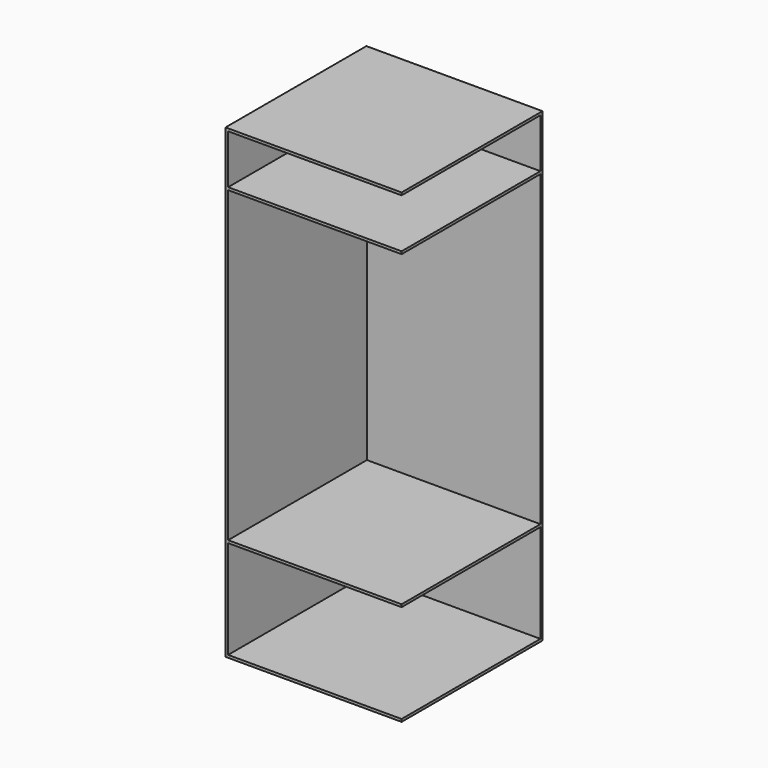
from build123d import *

# Parameters (mm, degrees)
F0_W        = 167.5
F0_H        = 85
F0_W_2      = 2.5
F0_H_2      = 2.5
F0_H_3      = 82.5
F1_DEPTH    = 100
F2_T        = -2.5
F3_W        = 2.5
F3_H        = 167.5
F3_W_2      = 167.5
F3_H_2      = 2.5
F4_DEPTH    = 300
F5_T        = 2.5
F5_T3_DEPTH = 172.5
F5_T5_DEPTH = 172.5
F5_T7_DEPTH = 100
F6_DEPTH    = 50
F7_T        = 2.5
F7_T3_DEPTH = 172.5
F7_T5_DEPTH = 172.5
F7_T7_DEPTH = 100
F7_T9_DEPTH = 302.5


# Not quite as in the source:
# - a shell that OpenCascade refuses in one call is made with other operations: the cavity is built on its own and cut out


with BuildPart() as f1:
    # F0 (on Top) → F1 (new body)
    with BuildSketch(Plane.XY):
        Polygon((82.5, -85), (85, -85), (85, 82.5), (82.5, 82.5), (82.5, 0), align=None)
        with Locations((-1.25, -42.5)):
            Rectangle(F0_W, F0_H)
        with Locations((83.75, 83.75)):
            Rectangle(F0_W_2, F0_H_2)
        with Locations((-1.25, 41.25)):
            Rectangle(F0_W, F0_H_3)
        with Locations((-1.25, 83.75)):
            Rectangle(F0_W, F0_H_2)
    extrude(amount=F1_DEPTH)

    # F2
    f2_openings = [f1.faces().sort_by_distance(p)[0] for p in [
        (85, 0, 50),
        (0, -85, 50),
    ]]
    offset(amount=F2_T, openings=f2_openings)

    # F3 (on face) → F4 (join)
    with BuildSketch(Plane.XY.offset(100)):
        with Locations((-83.75, -1.25)):
            Rectangle(F3_W, F3_H)
        with Locations((1.25, -1.25)):
            Rectangle(F3_W_2, F3_H)
        with Locations((-83.75, 83.75)):
            Rectangle(F3_W, F3_H_2)
        with Locations((1.25, 83.75)):
            Rectangle(F3_W_2, F3_H_2)
    extrude(amount=F4_DEPTH)

    # F5: shell of thickness 2.5, made by hand


with BuildPart() as f5_core1:
    # F5_t2: copy of F1
    add(f1.part)

    # the walls: a layer under each face that stays
    f5_faces = [f5_core1.faces().sort_by_distance(p)[0] for p in [
        (0, 85, 200),
        (0, 0, 0),
        (1.25, -1.25, 2.5),
        (1.25, 82.5, 50),
        (-82.5, -1.25, 50),
        (1.25, -1.25, 97.5),
        (-85, 0, 200),
        (0, 0, 400),
    ]]
    thicken(f5_faces, amount=-F5_T, mode=Mode.SUBTRACT)

    # F5_s4 → F5_t3 (cut)
    with BuildSketch(Plane.YZ.offset(-85)):
        Polygon((82.475, 2.525), (82.5, 0), (85, 0), (85, 2.5), align=None)
        Polygon((82.475, 97.475), (85, 97.5), (85, 100), (82.5, 100), align=None)
    extrude(amount=F5_T3_DEPTH, mode=Mode.SUBTRACT)

    # F5_s6 → F5_t5 (cut)
    with BuildSketch(Plane.XZ.offset(-85)):
        Polygon((-82.475, 2.525), (-82.5, 0), (-85, 0), (-85, 2.5), align=None)
        Polygon((-82.475, 97.475), (-85, 97.5), (-85, 100), (-82.5, 100), align=None)
    extrude(amount=F5_T5_DEPTH, mode=Mode.SUBTRACT)

    # F5_s8 → F5_t7 (cut)
    with BuildSketch(Plane.XY):
        Polygon((-82.475, 82.475), (-82.5, 85), (-85, 85), (-85, 82.5), align=None)
    extrude(amount=F5_T7_DEPTH, mode=Mode.SUBTRACT)


with BuildPart() as f1_1:
    add(f1.part)

    # what is left inside the walls is the cavity
    f5_cavity = [f5_core1.part.solids().sort_by_distance(p)[0] for p in [
        (1.25, 82.475, 298.333333),
    ]]
    add(f5_cavity, mode=Mode.SUBTRACT)

    # F6 (add): a face of the model
    f6_faces = [f1_1.faces().sort_by_distance(p)[0] for p in [
        (0, 0, 400),
    ]]
    extrude(f6_faces, amount=F6_DEPTH)

    # F7: shell of thickness 2.5, made by hand


with BuildPart() as f7_core1:
    # F7_t2: copy of F1
    add(f1_1.part)

    # the walls: a layer under each face that stays
    f7_faces = [f7_core1.faces().sort_by_distance(p)[0] for p in [
        (0, 85, 225),
        (0, 0, 0),
        (1.25, -1.25, 2.5),
        (1.25, 82.5, 50),
        (-82.5, -1.25, 50),
        (1.25, -1.25, 97.5),
        (1.25, -1.25, 100),
        (1.25, 82.5, 248.75),
        (-82.5, -1.25, 248.75),
        (1.25, -1.25, 397.5),
        (-85, 0, 225),
        (0, 0, 450),
    ]]
    thicken(f7_faces, amount=-F7_T, mode=Mode.SUBTRACT)

    # F7_s4 → F7_t3 (cut)
    with BuildSketch(Plane.YZ.offset(-85)):
        Polygon((82.475, 2.525), (82.5, 0), (85, 0), (85, 2.5), align=None)
        Polygon((82.475, 97.475), (85, 97.5), (85, 100), (82.5, 100), align=None)
        Polygon((82.475, 100.025), (82.5, 97.5), (85, 97.5), (85, 100), align=None)
        Polygon((82.475, 397.475), (85, 397.5), (85, 400), (82.5, 400), align=None)
    extrude(amount=F7_T3_DEPTH, mode=Mode.SUBTRACT)

    # F7_s6 → F7_t5 (cut)
    with BuildSketch(Plane.XZ.offset(-85)):
        Polygon((-82.475, 2.525), (-82.5, 0), (-85, 0), (-85, 2.5), align=None)
        Polygon((-82.475, 97.475), (-85, 97.5), (-85, 100), (-82.5, 100), align=None)
        Polygon((-82.475, 100.025), (-82.5, 97.5), (-85, 97.5), (-85, 100), align=None)
        Polygon((-82.475, 397.475), (-85, 397.5), (-85, 400), (-82.5, 400), align=None)
    extrude(amount=F7_T5_DEPTH, mode=Mode.SUBTRACT)

    # F7_s8 → F7_t7 (cut)
    with BuildSketch(Plane.XY):
        Polygon((-82.475, 82.475), (-82.5, 85), (-85, 85), (-85, 82.5), align=None)
    extrude(amount=F7_T7_DEPTH, mode=Mode.SUBTRACT)

    # F7_s10 → F7_t9 (cut)
    with BuildSketch(Plane.XY.offset(97.5)):
        Polygon((-82.475, 82.475), (-82.5, 85), (-85, 85), (-85, 82.5), align=None)
    extrude(amount=F7_T9_DEPTH, mode=Mode.SUBTRACT)


with BuildPart() as f1_2:
    add(f1_1.part)

    # what is left inside the walls is the cavity
    f7_cavity = [f7_core1.part.solids().sort_by_distance(p)[0] for p in [
        (1.25, -29.166667, 447.475),
    ]]
    add(f7_cavity, mode=Mode.SUBTRACT)


solid = f1_2.part
